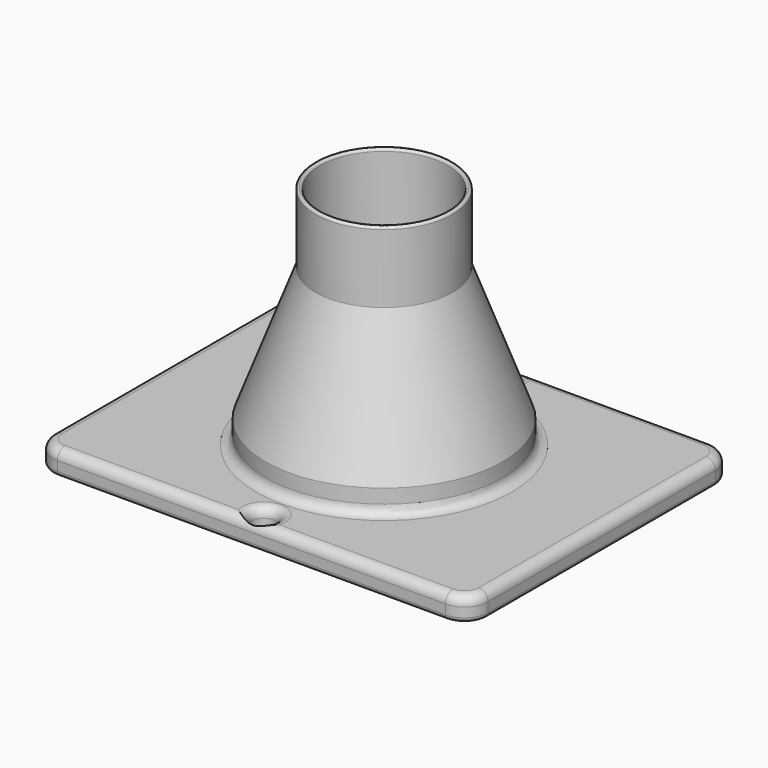
from build123d import *

# Parameters (mm, degrees)
F3_W          = 92
F3_H          = 70
F3_R          = 2.5
F4_DEPTH      = 5
F5_R          = 23.5
F6_DEPTH      = 5
F7_T3_DEPTH   = 102
F7_T5_DEPTH   = 80
F8_T1_DEPTH   = 17.4999999999
F8_T4_ANGLE   = 90
F8_T6_ANGLE   = 90
F8_T8_ANGLE   = 90
F8_T10_ANGLE  = 90
F9_R          = 0.49999
F10_T1_DEPTH  = 60
F10_T3_DEPTH  = 82
F10_T6_ANGLE  = 89.9999999974
F10_T8_ANGLE  = 89.9999999974
F10_T10_ANGLE = 89.9999999974
F10_T12_ANGLE = 89.9999999974


# Not quite as in the source:
# - a fillet or chamfer that OpenCascade refuses, or shapes differently, is made with other operations: its cross-section is extruded or revolved along the edge and cut away or added
# - a fillet or chamfer is up to 0.001 mm smaller than in the source, because OpenCascade refuses the exact size


with BuildPart() as f1:
    # F0 (on Front) → F1 (revolve)
    with BuildSketch(Plane.XZ):
        Polygon((-25, 10), (-25, 0), (-24, 0), (-24, 9.8192848565), (-13.5, 37.9217758492), (-13.5, 53.1024909928), (-14.5, 53.1024909928), (-14.5, 38.1024909928), align=None)
    revolve(axis=Axis((0, 0, 23.4480407089), (0, 0, 1)))

    # F3 (on offset) → F4 (join)
    with BuildSketch(Plane(origin=(0, 0, 0), x_dir=(1, 0, 0), z_dir=(0, 0, -1))):
        Rectangle(F3_W, F3_H)
        with Locations((0, -31.75)):
            Circle(F3_R, mode=Mode.SUBTRACT)
        with Locations((0, 31.75)):
            Circle(F3_R, mode=Mode.SUBTRACT)
    extrude(amount=-F4_DEPTH)

    # F5 (on face) → F6 (cut, through all)
    with BuildSketch(Plane(origin=(0, 0, 0), x_dir=(1, 0, 0), z_dir=(0, 0, -1))):
        Circle(F5_R)
    extrude(amount=-F6_DEPTH, mode=Mode.SUBTRACT)

    # F7: fillet of radius 2 on 7 edges, made by hand

    # F7_s1 → F7_t2 (revolve)
    with BuildSketch(Plane.XZ):
        with BuildLine():
            ThreePointArc((-25, 7), (-25.5857864376, 5.5857864376), (-27, 5))
            Line((-27, 5), (-25, 5))
            Line((-25, 5), (-25, 7))
        make_face()
    revolve(axis=Axis((0, 0, 5), (0, 0, -1)))

    # F7_s4 → F7_t3 (cut)
    with BuildSketch(Plane.YZ.offset(-51)):
        with BuildLine():
            ThreePointArc((-33, 5), (-34.4142135624, 4.4142135624), (-35, 3))
            Line((-35, 3), (-35, 5))
            Line((-35, 5), (-33, 5))
        make_face()
        with BuildLine():
            ThreePointArc((33, 5), (34.4142135624, 4.4142135624), (35, 3))
            Line((35, 3), (35, 5))
            Line((35, 5), (33, 5))
        make_face()
    extrude(amount=F7_T3_DEPTH, mode=Mode.SUBTRACT)

    # F7_s6 → F7_t5 (cut)
    with BuildSketch(Plane.XZ.offset(-40)):
        with BuildLine():
            ThreePointArc((44, 5), (45.4142135624, 4.4142135624), (46, 3))
            Line((46, 3), (46, 5))
            Line((46, 5), (44, 5))
        make_face()
        with BuildLine():
            ThreePointArc((-44, 5), (-45.4142135624, 4.4142135624), (-46, 3))
            Line((-46, 3), (-46, 5))
            Line((-46, 5), (-44, 5))
        make_face()
    extrude(amount=F7_T5_DEPTH, mode=Mode.SUBTRACT)

    # F7_s7 → F7_t8 (revolve, cut)
    with BuildSketch(Plane.XZ.offset(-31.75)):
        with BuildLine():
            ThreePointArc((4.5, 5), (3.0857864376, 4.4142135624), (2.5, 3))
            Line((2.5, 3), (2.5, 5))
            Line((2.5, 5), (4.5, 5))
        make_face()
    revolve(axis=Axis((0, 31.75, 5), (0, 0, -1)), mode=Mode.SUBTRACT)

    # F7_s9 → F7_t10 (revolve, cut)
    with BuildSketch(Plane.XZ.offset(31.75)):
        with BuildLine():
            ThreePointArc((4.5, 5), (3.0857864376, 4.4142135624), (2.5, 3))
            Line((2.5, 3), (2.5, 5))
            Line((2.5, 5), (4.5, 5))
        make_face()
    revolve(axis=Axis((0, -31.75, 5), (0, 0, -1)), mode=Mode.SUBTRACT)

    # F8: fillet of radius 5 on 4 edges, made by hand

    # F8_s2 → F8_t1 (cut)
    with BuildSketch(Plane.XY.offset(-12.5)):
        with BuildLine():
            ThreePointArc((41, -35), (44.5355339059, -33.5355339059), (46, -30))
            Line((46, -30), (46, -35))
            Line((46, -35), (41, -35))
        make_face()
        with BuildLine():
            ThreePointArc((-46, -30), (-44.5355339059, -33.5355339059), (-41, -35))
            Line((-41, -35), (-46, -35))
            Line((-46, -35), (-46, -30))
        make_face()
        with BuildLine():
            ThreePointArc((-41, 35), (-44.5355339059, 33.5355339059), (-46, 30))
            Line((-46, 30), (-46, 35))
            Line((-46, 35), (-41, 35))
        make_face()
        with BuildLine():
            ThreePointArc((41, 35), (44.5355339059, 33.5355339059), (46, 30))
            Line((46, 30), (46, 35))
            Line((46, 35), (41, 35))
        make_face()
    extrude(amount=F8_T1_DEPTH, mode=Mode.SUBTRACT)

    # F8_s3 → F8_t4 (revolve, cut)
    with BuildSketch(Plane.XZ.offset(-30)):
        with BuildLine():
            ThreePointArc((44.0000000001, 5), (45.4142135624, 4.4142135624), (46, 3.0000000001))
            Line((46, 3.0000000001), (46, 5))
            Line((46, 5), (44.0000000001, 5))
        make_face()
    revolve(axis=Axis((41, 30, 5), (0, 0, 1)), revolution_arc=F8_T4_ANGLE, mode=Mode.SUBTRACT)

    # F8_s5 → F8_t6 (revolve, cut)
    with BuildSketch(Plane.YZ.offset(-41)):
        with BuildLine():
            ThreePointArc((33.0000000001, 5), (34.4142135624, 4.4142135624), (35, 3.0000000001))
            Line((35, 3.0000000001), (35, 5))
            Line((35, 5), (33.0000000001, 5))
        make_face()
    revolve(axis=Axis((-41, 30, 5), (0, 0, 1)), revolution_arc=F8_T6_ANGLE, mode=Mode.SUBTRACT)

    # F8_s7 → F8_t8 (revolve, cut)
    with BuildSketch(Plane.XZ.offset(30)):
        with BuildLine():
            ThreePointArc((-44.0000000001, 5), (-45.4142135624, 4.4142135624), (-46, 3.0000000001))
            Line((-46, 3.0000000001), (-46, 5))
            Line((-46, 5), (-44.0000000001, 5))
        make_face()
    revolve(axis=Axis((-41, -30, 5), (0, 0, 1)), revolution_arc=F8_T8_ANGLE, mode=Mode.SUBTRACT)

    # F8_s9 → F8_t10 (revolve, cut)
    with BuildSketch(Plane.YZ.offset(41)):
        with BuildLine():
            ThreePointArc((-33.0000000001, 5), (-34.4142135624, 4.4142135624), (-35, 3.0000000001))
            Line((-35, 3.0000000001), (-35, 5))
            Line((-35, 5), (-33.0000000001, 5))
        make_face()
    revolve(axis=Axis((41, -30, 5), (0, 0, 1)), revolution_arc=F8_T10_ANGLE, mode=Mode.SUBTRACT)

    # F9 (radius 0.5 in the source; OpenCascade refuses exactly that, so slightly less here)
    f9_edges = [f1.edges().sort_by_distance(p)[0] for p in [
        (13.5, 0, 53.102491),
        (14.5, 0, 53.102491),
    ]]
    fillet(f9_edges, radius=F9_R)

    # F10: fillet of radius 1 on 11 edges, made by hand

    # F10_s2 → F10_t1 (cut)
    with BuildSketch(Plane.XZ.offset(-30)):
        with BuildLine():
            ThreePointArc((46, 1), (45.7071067812, 0.2928932188), (45, 0))
            Line((45, 0), (46, 0))
            Line((46, 0), (46, 1))
        make_face()
        with BuildLine():
            ThreePointArc((-46, 1), (-45.7071067812, 0.2928932188), (-45, 0))
            Line((-45, 0), (-46, 0))
            Line((-46, 0), (-46, 1))
        make_face()
    extrude(amount=F10_T1_DEPTH, mode=Mode.SUBTRACT)

    # F10_s4 → F10_t3 (cut)
    with BuildSketch(Plane.YZ.offset(-41)):
        with BuildLine():
            ThreePointArc((35, 1), (34.7071067812, 0.2928932188), (34, 0))
            Line((34, 0), (35, 0))
            Line((35, 0), (35, 1))
        make_face()
        with BuildLine():
            ThreePointArc((-35, 1), (-34.7071067812, 0.2928932188), (-34, 0))
            Line((-34, 0), (-35, 0))
            Line((-35, 0), (-35, 1))
        make_face()
    extrude(amount=F10_T3_DEPTH, mode=Mode.SUBTRACT)

    # F10_s5 → F10_t6 (revolve, cut)
    with BuildSketch(Plane.XZ.offset(29.9999999999)):
        with BuildLine():
            ThreePointArc((46, 1), (45.7071067812, 0.2928932188), (45, 0))
            Line((45, 0), (46, 0))
            Line((46, 0), (46, 1))
        make_face()
    revolve(axis=Axis((40.9999999999, -29.9999999999, 0), (0, 0, -1)), revolution_arc=F10_T6_ANGLE, mode=Mode.SUBTRACT)

    # F10_s7 → F10_t8 (revolve, cut)
    with BuildSketch(Plane.YZ.offset(40.9999999999)):
        with BuildLine():
            ThreePointArc((35, 1), (34.7071067812, 0.2928932188), (34, 0))
            Line((34, 0), (35, 0))
            Line((35, 0), (35, 1))
        make_face()
    revolve(axis=Axis((40.9999999999, 29.9999999999, 0), (0, 0, -1)), revolution_arc=F10_T8_ANGLE, mode=Mode.SUBTRACT)

    # F10_s9 → F10_t10 (revolve, cut)
    with BuildSketch(Plane.XZ.offset(-29.9999999999)):
        with BuildLine():
            ThreePointArc((-46, 1), (-45.7071067812, 0.2928932188), (-45, 0))
            Line((-45, 0), (-46, 0))
            Line((-46, 0), (-46, 1))
        make_face()
    revolve(axis=Axis((-40.9999999999, 29.9999999999, 0), (0, 0, -1)), revolution_arc=F10_T10_ANGLE, mode=Mode.SUBTRACT)

    # F10_s11 → F10_t12 (revolve, cut)
    with BuildSketch(Plane.YZ.offset(-40.9999999999)):
        with BuildLine():
            ThreePointArc((-35, 1), (-34.7071067812, 0.2928932188), (-34, 0))
            Line((-34, 0), (-35, 0))
            Line((-35, 0), (-35, 1))
        make_face()
    revolve(axis=Axis((-40.9999999999, -29.9999999999, 0), (0, 0, -1)), revolution_arc=F10_T12_ANGLE, mode=Mode.SUBTRACT)

    # F10_s13 → F10_t14 (revolve, cut)
    with BuildSketch(Plane.XZ.offset(-31.75)):
        with BuildLine():
            ThreePointArc((2.5, 1), (2.7928932188, 0.2928932188), (3.5, 0))
            Line((3.5, 0), (2.5, 0))
            Line((2.5, 0), (2.5, 1))
        make_face()
    revolve(axis=Axis((0, 31.75, 0), (0, 0, -1)), mode=Mode.SUBTRACT)

    # F10_s15 → F10_t16 (revolve, cut)
    with BuildSketch(Plane.XZ):
        with BuildLine():
            ThreePointArc((24.5, 0), (23.7928932188, 0.2928932188), (23.5, 1))
            Line((23.5, 1), (23.5, 0))
            Line((23.5, 0), (24.5, 0))
        make_face()
    revolve(axis=Axis((0, 0, 0), (0, 0, -1)), mode=Mode.SUBTRACT)

    # F10_s17 → F10_t18 (revolve, cut)
    with BuildSketch(Plane.XZ.offset(31.75)):
        with BuildLine():
            ThreePointArc((2.5, 1), (2.7928932188, 0.2928932188), (3.5, 0))
            Line((3.5, 0), (2.5, 0))
            Line((2.5, 0), (2.5, 1))
        make_face()
    revolve(axis=Axis((0, -31.75, 0), (0, 0, -1)), mode=Mode.SUBTRACT)


solid = f1.part
